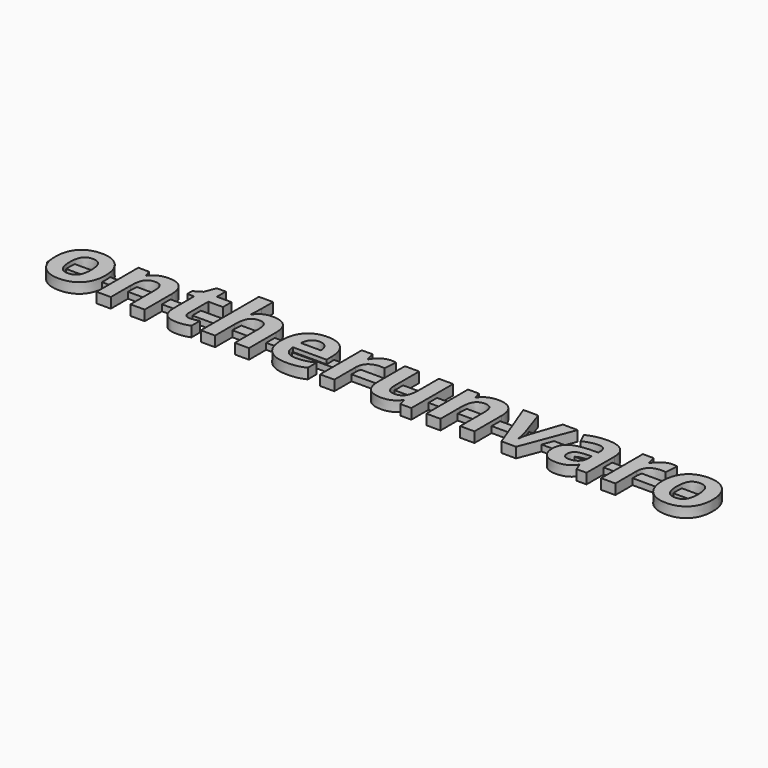
from build123d import *

# Parameters (mm, degrees)
F0_TEXT_SIZE = 9.2950508323
F1_DEPTH     = 1
F2_W         = 64.0599653125
F2_H         = 1.0341410525
F3_DEPTH     = 0.6


# Not quite as in the source:
# - Text() gives the source's letters only with a copy of the font that has no kerning and outlines rounded to 1/6400 em; it was checked with that copy


with BuildPart() as f1:
    # F0 (on Top) → F1 (new body)
    with BuildSketch(Plane.XY):
        with Locations((0, -6.6924365993)):
            Text('ontherunvaro', F0_TEXT_SIZE, font='Open Sans', font_style=FontStyle.BOLD, text_align=(TextAlign.LEFT, TextAlign.BOTTOM))
    extrude(amount=F1_DEPTH)

    # F2 (on Top) → F3 (join)
    with BuildSketch(Plane.XY):
        with Locations((32.0299826562, -4.0809281636)):
            Rectangle(F2_W, F2_H)
    extrude(amount=F3_DEPTH)


solid = f1.part
